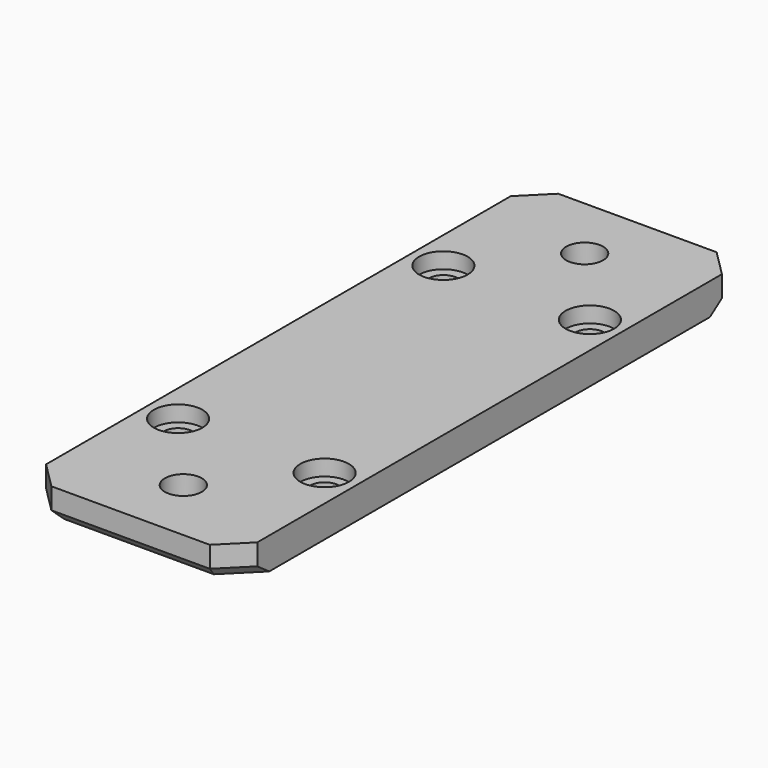
from build123d import *

# Parameters (mm, degrees)
F0_W           = 40
F0_H           = 120
F1_DEPTH       = 6
F3_D           = 5.5
F3_DEPTH       = 15
F3_CBORE_D     = 9.2
F3_CBORE_DEPTH = 3
F3_TIP         = 1.6523667023
F5_D           = 7
F5_DEPTH       = 15
F5_TIP         = 2.1030121666
F6_SIZE        = 5
F7_SIZE        = 2


# Not quite as in the source:
# - a pattern or mirror of a feature is missing from the dataset's text; its kind, count and spacing are read off the source's solid


with BuildPart() as f1:
    # F0 (on Top) → F1 (new body)
    with BuildSketch(Plane.XY):
        Rectangle(F0_W, F0_H)
    extrude(amount=F1_DEPTH)

    # F3
    with Locations(Plane.XY.offset(6)):
        with Locations((-13.875, 31.4), (13.875, 31.4), (-13.875, -31.4), (13.875, -31.4)):
            CounterBoreHole(F3_D / 2, F3_CBORE_D / 2, F3_CBORE_DEPTH, depth=F3_DEPTH)
            with Locations((0, 0, -(F3_DEPTH + F3_TIP / 2))):  # 118° drill point
                Cone(0, F3_D / 2, F3_TIP, mode=Mode.SUBTRACT)

    # F5
    with Locations(Plane.XY.offset(6)):
        with Locations((0, 47.5)):
            f5 = Hole(F5_D / 2, depth=F5_DEPTH)
            with Locations((0, 0, -(F5_DEPTH + F5_TIP / 2))):  # 118° drill point
                Cone(0, F5_D / 2, F5_TIP, mode=Mode.SUBTRACT)

    # F5_copies: F5 across plane
    add(f5.mirror(Plane(origin=(0, 0, 0), x_dir=(0, 0, -1), z_dir=(0, -1, 0))), mode=Mode.SUBTRACT)

    # F6
    f6_edges = [f1.edges().sort_by_distance(p)[0] for p in [
        (20, 60, 3),
        (-20, 60, 3),
        (-20, -60, 3),
        (20, -60, 3),
    ]]
    chamfer(f6_edges, length=F6_SIZE)

    # F7
    f7_edges = [f1.edges().sort_by_distance(p)[0] for p in [
        (0, 60, 0),
        (-17.5, 57.5, 0),
        (17.5, 57.5, 0),
        (17.5, -57.5, 0),
        (0, -60, 0),
        (-17.5, -57.5, 0),
    ]]
    chamfer(f7_edges, length=F7_SIZE)


solid = f1.part
